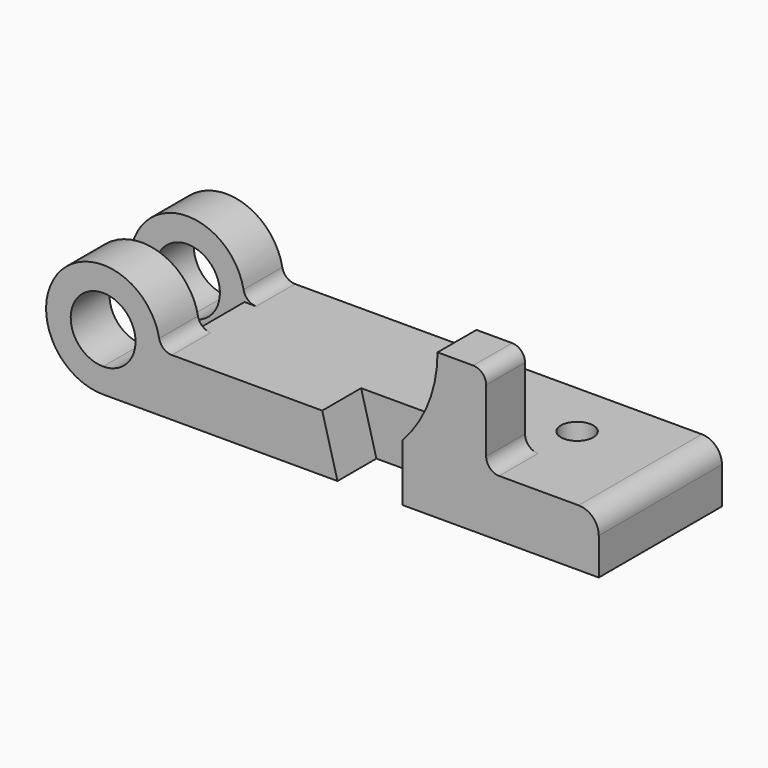
from build123d import *

# Parameters (mm, degrees)
F1_DEPTH = 30.1625
F2_DEPTH = 11.1633
F4_DEPTH = 19.05
F5_DEPTH = 19.05
F6_R     = 7.874
F7_R     = 5.08
F8_R     = 6.35
F9_DEPTH = 22.353


with BuildPart() as f1:
    # F0 (on Front) → F1 (new body, symmetric)
    with BuildSketch(Plane.XZ):
        Polygon((97.8408, -22.352), (117.2485877871, -22.352), (117.2485877871, 0), (91.8464, 0), align=None)
        Polygon((91.8464, -22.352), (91.8464, 0), (85.852, 0), align=None)
        Polygon((64.8810639977, -22.352), (91.8464, -22.352), (85.852, 0), (43.9732931554, 0), align=None)
        with BuildLine():
            Line((0, -22.352), (64.8810639977, -22.352))
            Line((64.8810639977, -22.352), (43.9732931554, 0))
            Line((43.9732931554, 0), (22.352, 0))
            ThreePointArc((22.352, 0), (15.8052507731, -15.8052507731), (0, -22.352))
        make_face()
        with BuildLine():
            ThreePointArc((22.352, 0), (-15.8052507731, 15.8052507731), (0, -22.352))
            Line((0, -22.352), (0, -12.7))
            ThreePointArc((0, -12.7), (-8.9802561211, 8.9802561211), (12.7, 0))
            Line((12.7, 0), (22.352, 0))
        make_face()
        Polygon((91.8464, -22.352), (97.8408, -22.352), (91.8464, 0), align=None)
        Polygon((194.2084, -22.352), (194.2084, 0), (150.0886, 0), (131.0386, 0), (117.2485877871, 0), (117.2485877871, -22.352), align=None)
        with BuildLine():
            Line((0, -12.7), (0, -22.352))
            ThreePointArc((0, -22.352), (15.8052507731, -15.8052507731), (22.352, 0))
            Line((22.352, 0), (12.7, 0))
            ThreePointArc((12.7, 0), (8.9802561211, -8.9802561211), (0, -12.7))
        make_face()
    extrude(amount=F1_DEPTH, both=True)

    # F0 (on Front) → F2 (cut, symmetric)
    with BuildSketch(Plane.XZ):
        with BuildLine():
            ThreePointArc((22.352, 0), (-15.8052507731, 15.8052507731), (0, -22.352))
            Line((0, -22.352), (0, -12.7))
            ThreePointArc((0, -12.7), (-8.9802561211, 8.9802561211), (12.7, 0))
            Line((12.7, 0), (22.352, 0))
        make_face()
        with BuildLine():
            Line((0, -12.7), (0, -22.352))
            ThreePointArc((0, -22.352), (15.8052507731, -15.8052507731), (22.352, 0))
            Line((22.352, 0), (12.7, 0))
            ThreePointArc((12.7, 0), (8.9802561211, -8.9802561211), (0, -12.7))
        make_face()
    extrude(amount=F2_DEPTH, both=True, mode=Mode.SUBTRACT)

    # F3 (on face) → F4 (cut)
    with BuildSketch(Plane.XZ.offset(30.1625)):
        Polygon((117.2485877871, -22.352), (117.2485877871, 0), (85.852, 0), (91.8464, -22.352), align=None)
    extrude(amount=-F4_DEPTH, mode=Mode.SUBTRACT)

    # F3 (on face) → F5 (join)
    with BuildSketch(Plane.XZ.offset(30.1625)):
        with BuildLine():
            ThreePointArc((131.0386, 34.798), (127.4654323074, 16.0825969798), (117.2485877871, 0))
            Line((117.2485877871, 0), (150.0886, 0))
            Line((150.0886, 0), (150.0886, 34.798))
            Line((150.0886, 34.798), (131.0386, 34.798))
        make_face()
    extrude(amount=-F5_DEPTH)

    # F6
    f6_edges = [f1.edges().sort_by_distance(p)[0] for p in [
        (194.2084, 0, 0),
    ]]
    fillet(f6_edges, radius=F6_R)

    # F7
    f7_edges = [f1.edges().sort_by_distance(p)[0] for p in [
        (150.0886, -20.6375, 34.798),
        (150.0886, -20.6375, 0),
        (22.352, 20.6629, 0),
        (22.352, -20.6629, 0),
    ]]
    fillet(f7_edges, radius=F7_R)

    # F8 (on face) → F9 (cut, through all)
    with BuildSketch(Plane.XY):
        with Locations((155.3464, 7.8105)):
            Circle(F8_R)
    extrude(amount=-F9_DEPTH, mode=Mode.SUBTRACT)


solid = f1.part
